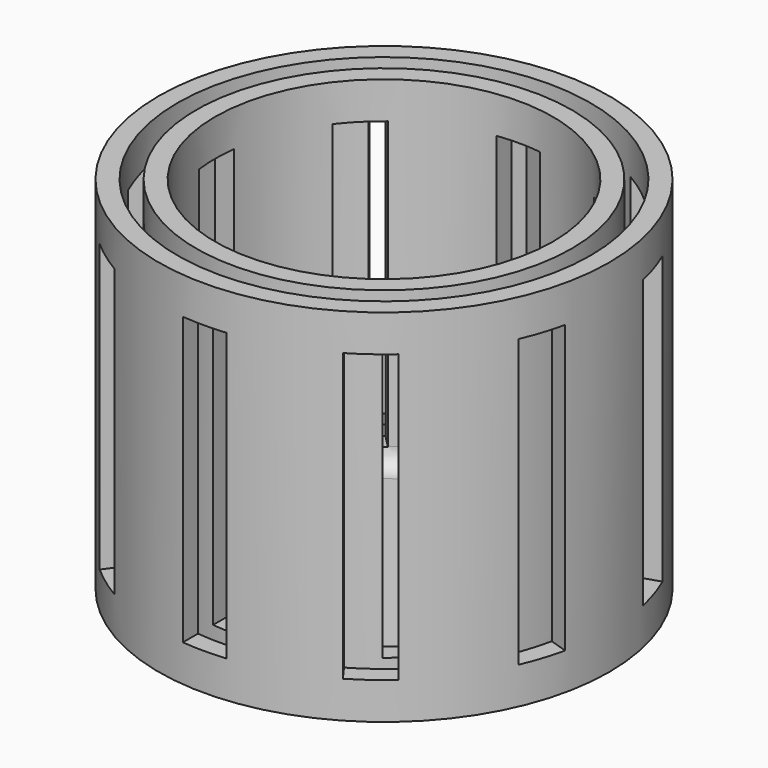
from build123d import *

# Parameters (mm, degrees)
F2_W            = 11.5754483268
F2_H            = 76.3443418741
F3_REACH        = 137.2178993172
F3_COPIES_COUNT = 8
F5_W            = 11.5754483268
F5_H            = 76.3443418741
F6_REACH        = 212.2178993172
F6_COPIES_COUNT = 10


# Not quite as in the source:
# - a pattern or mirror of a feature is missing from the dataset's text; its kind, count and spacing are read off the source's solid


with BuildPart() as f1:
    # F0 (on Front) → F1 (revolve)
    with BuildSketch(Plane.XZ):
        with BuildLine():
            Line((0, 5), (0, 0))
            Line((0, 0), (60, 0))
            Line((60, 0), (60, 96))
            Line((60, 96), (55, 96))
            Line((55, 96), (55, 5))
            Line((55, 5), (50, 5))
            Line((50, 5), (50, 96))
            Line((50, 96), (45, 96))
            Line((45, 96), (45, 10))
            ThreePointArc((45, 10), (43.5355339059, 6.4644660941), (40, 5))
            Line((40, 5), (0, 5))
        make_face()
    revolve(axis=Axis((0, 0, 2.5), (0, 0, 1)))

    f3_end = f1.faces().sort_by_distance((-50, 0, 50.5))[0]
    # F2 (on Front) → F3 (cut, up to a face of the model that its end follows)
    with BuildSketch(Plane.XZ):
        with Locations((0, 48)):
            Rectangle(F2_W, F2_H)
    f3_long = extrude(amount=F3_REACH, mode=Mode.PRIVATE)
    f3 = split(f3_long, bisect_by=f3_end, keep=Keep.BOTTOM, mode=Mode.PRIVATE)
    add(f3, mode=Mode.SUBTRACT)

    # F3_copies: F3 ×8 about axis
    f3_copies_axis = Axis((0, 0, 0), (0, 0, 1))
    for i in range(1, F3_COPIES_COUNT):
        add(f3.rotate(f3_copies_axis, i * 360 / F3_COPIES_COUNT), mode=Mode.SUBTRACT)

    f6_end = f1.faces().sort_by_distance((-55, 0, 50.5))[0]
    # F5 (on offset) → F6 (cut, up to a face of the model that its end follows)
    with BuildSketch(Plane.XZ.offset(75)):
        with Locations((0, 48)):
            Rectangle(F5_W, F5_H)
    f6_long = extrude(amount=-F6_REACH, mode=Mode.PRIVATE)
    f6 = split(f6_long, bisect_by=f6_end, keep=Keep.ALL, mode=Mode.PRIVATE).solids().sort_by_distance((0, -75, 48))[0]
    add(f6, mode=Mode.SUBTRACT)

    # F6_copies: F6 ×10 about axis
    f6_copies_axis = Axis((0, 0, 0), (0, 0, 1))
    for i in range(1, F6_COPIES_COUNT):
        add(f6.rotate(f6_copies_axis, i * 360 / F6_COPIES_COUNT), mode=Mode.SUBTRACT)


solid = f1.part
